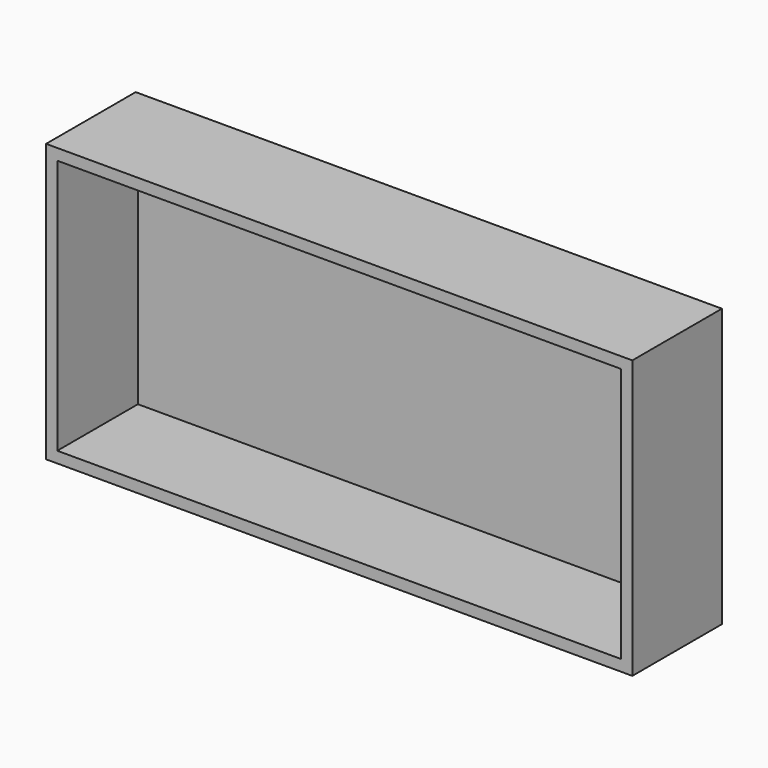
from build123d import *

# Parameters (mm, degrees)
F0_W     = 132.97829777
F0_H     = 63.0043921992
F1_DEPTH = 25.4
F2_T     = -2.54


# Not quite as in the source:
# - a feature of the source that left no trace in its solid (it failed there, or was rolled back) is left out


with BuildPart() as f1:
    # F0 (on Front) → F1 (new body)
    with BuildSketch(Plane.XZ):
        with Locations((-9.4785355031, 24.2539034225)):
            Rectangle(F0_W, F0_H)
    extrude(amount=F1_DEPTH)

    # F2
    f2_openings = [f1.faces().sort_by_distance(p)[0] for p in [
        (-9.478536, -25.4, 24.253903),
    ]]
    offset(amount=F2_T, openings=f2_openings)


solid = f1.part
